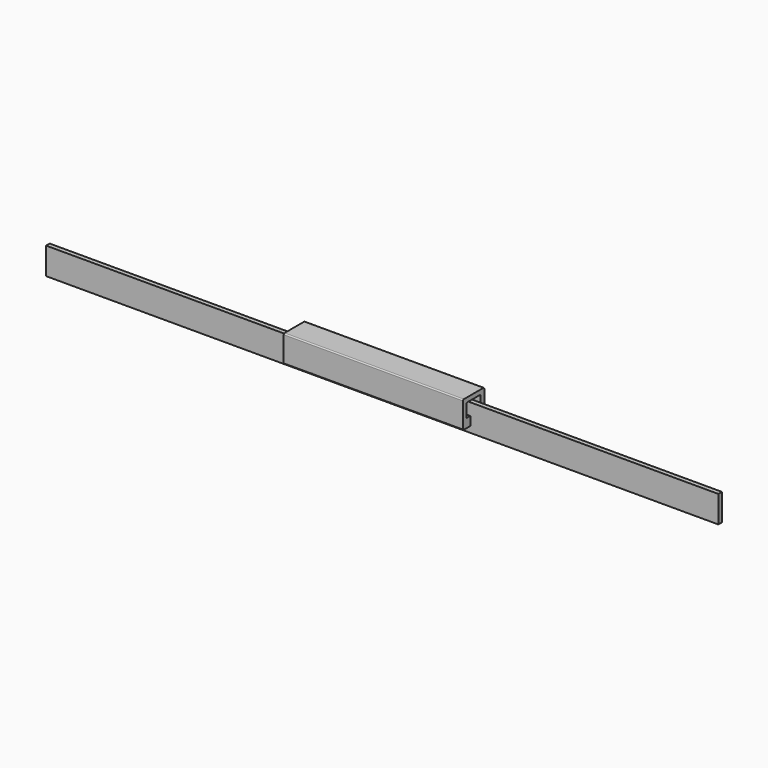
from build123d import *

# Parameters (mm, degrees)
F0_W     = 2
F0_H     = 12
F1_DEPTH = 150
F5_DEPTH = 40


# Not quite as in the source:
# - the program builds the solid bodies; features that only make, move or delete a surface that nothing else refers to are left out


with BuildPart() as f1:
    # F0 (on Right) → F1 (new body, symmetric)
    with BuildSketch(Plane.YZ):
        Rectangle(F0_W, F0_H)
    extrude(amount=F1_DEPTH, both=True)


with BuildPart() as f5:
    # F4 (on Right) → F5 (new body, symmetric)
    with BuildSketch(Plane.YZ):
        with BuildLine():
            ThreePointArc((-1.6229878874, 0.7658509659), (-1.7694344968, 1.1194043565), (-2.1229878874, 1.2658509659))
            Line((-2.1229878874, 1.2658509659), (-3.9153032975, 1.2658509659))
            Line((-3.9153032975, 1.2658509659), (-3.9153032975, 6.7658509659))
            ThreePointArc((-3.9153032975, 6.7658509659), (-3.7688566881, 7.1194043565), (-3.4153032975, 7.2658509659))
            Line((-3.4153032975, 7.2658509659), (3.4153032975, 7.2658509659))
            ThreePointArc((3.4153032975, 7.2658509659), (3.7688566881, 7.1194043565), (3.9153032975, 6.7658509659))
            Line((3.9153032975, 6.7658509659), (3.9153032975, 1.2658509659))
            Line((3.9153032975, 1.2658509659), (1.7367364252, 1.2658509659))
            ThreePointArc((1.7367364252, 1.2658509659), (1.3831830346, 1.1194043565), (1.2367364252, 0.7658509659))
            Line((1.2367364252, 0.7658509659), (1.2367364252, -2.7341490341))
            Line((1.2367364252, -2.7341490341), (5.4347978226, -2.7341490341))
            ThreePointArc((5.4347978226, -2.7341490341), (5.7883512131, -2.5877024247), (5.9347978226, -2.2341490341))
            Line((5.9347978226, -2.2341490341), (5.9347978226, 8.7658509659))
            ThreePointArc((5.9347978226, 8.7658509659), (5.7883512131, 9.1194043565), (5.4347978226, 9.2658509659))
            Line((5.4347978226, 9.2658509659), (-5.4347978226, 9.2658509659))
            ThreePointArc((-5.4347978226, 9.2658509659), (-5.7883512131, 9.1194043565), (-5.9347978226, 8.7658509659))
            Line((-5.9347978226, 8.7658509659), (-5.9347978226, -2.2341490341))
            ThreePointArc((-5.9347978226, -2.2341490341), (-5.7883512131, -2.5877024247), (-5.4347978226, -2.7341490341))
            Line((-5.4347978226, -2.7341490341), (-2.1229878874, -2.7341490341))
            ThreePointArc((-2.1229878874, -2.7341490341), (-1.7694344968, -2.5877024247), (-1.6229878874, -2.2341490341))
            Line((-1.6229878874, -2.2341490341), (-1.6229878874, 0.7658509659))
        make_face()
    extrude(amount=F5_DEPTH, both=True)


with BuildPart() as f6_1:
    # F6: copy of F5
    add(f5.part)


solid = Compound([f1.part, f5.part, f6_1.part])
